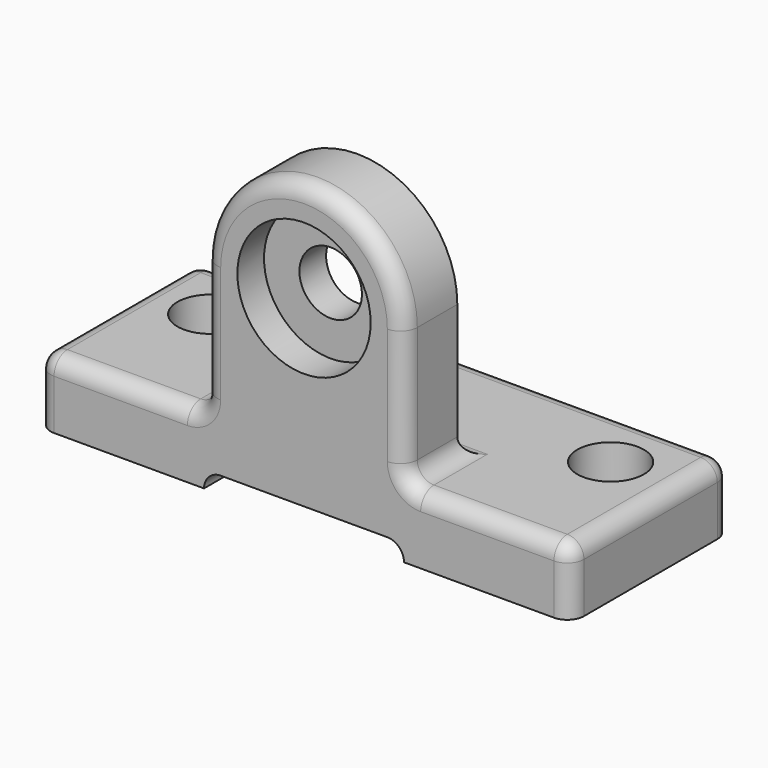
from build123d import *

# Parameters (mm, degrees)
F0_W           = 101.6
F0_H           = 38.1
F0_R           = 6.35
F1_DEPTH       = 12.7
F3_DEPTH       = 12.7
F4_D           = 11.90625
F4_CBORE_D     = 25.4
F4_CBORE_DEPTH = 6.35
F5_W           = 38.1
F5_H           = 3.175
F6_DEPTH       = 38.101
F9_R           = 3.175
F9_R_2         = 3.17499


# Not quite as in the source:
# - a fillet or chamfer is up to 0.001 mm smaller than in the source, because OpenCascade refuses the exact size
# - a feature of the source that left no trace in its solid (it failed there, or was rolled back) is left out
# - a length typed as a fraction of an inch, garbled in the dataset ("3 / 203.2 mm" for 3/8 in), is restored


with BuildPart() as f1:
    # F0 (on Top) → F1 (new body)
    with BuildSketch(Plane.XY):
        with Locations((12.3613710271, 3.3725141548)):
            Rectangle(F0_W, F0_H)
        with Locations((-25.7386289729, 9.7225141548)):
            Circle(F0_R, mode=Mode.SUBTRACT)
        with Locations((50.4613710271, 9.7225141548)):
            Circle(F0_R, mode=Mode.SUBTRACT)
    extrude(amount=F1_DEPTH)

    # F2 (on face) → F3 (join)
    with BuildSketch(Plane.XZ.offset(15.6774858452)):
        with BuildLine():
            Line((-6.6886289729, 38.1), (-6.6886289729, 12.7))
            Line((-6.6886289729, 12.7), (31.4113710271, 12.7))
            Line((31.4113710271, 12.7), (31.4113710271, 38.1))
            ThreePointArc((31.4113710271, 38.1), (12.3613710271, 57.15), (-6.6886289729, 38.1))
        make_face()
    extrude(amount=-F3_DEPTH)

    # F4 (through all)
    with Locations(Plane.XZ.offset(15.6774858452)):
        with Locations((12.3613710271, 38.1)):
            CounterBoreHole(F4_D / 2, F4_CBORE_D / 2, F4_CBORE_DEPTH)

    # F5 (on face) → F6 (cut, through all)
    with BuildSketch(Plane(origin=(0, 22.4225141548, 0), x_dir=(-1, 0, 0), z_dir=(0, 1, 0))):
        with Locations((-12.3613710271, 1.5875)):
            Rectangle(F5_W, F5_H)
    extrude(amount=-F6_DEPTH, mode=Mode.SUBTRACT)

    # F8: union 

    # F9 (call 1 of 3: OpenCascade refuses the feature's edges together)
    f9_edges = [f1.edges().sort_by_distance(p)[0] for p in [
        (63.161371, -15.677486, 6.35),
        (63.161371, 22.422514, 6.35),
        (-38.438629, -15.677486, 6.35),
        (-38.438629, 22.422514, 6.35),
        (12.361371, 22.422514, 12.7),
        (63.161371, 3.372514, 12.7),
        (-38.438629, 3.372514, 12.7),
        (47.286371, -15.677486, 12.7),
        (-22.563629, -15.677486, 12.7),
        (12.361371, -2.977486, 12.7),
        (31.411371, -9.327486, 12.7),
        (-6.688629, -9.327486, 12.7),
        (31.411371, -15.677486, 25.4),
        (12.361371, -15.677486, 57.15),
        (-6.688629, -15.677486, 25.4),
    ]]
    fillet(f9_edges, radius=F9_R)

    # F9#2 (call 2 of 3) (radius 3.175 in the source; OpenCascade refuses exactly that, so slightly less here)
    f9_2_edges = [f1.edges().sort_by_distance(p)[0] for p in [
        (-6.688629, 3.372514, 3.175),
    ]]
    fillet(f9_2_edges, radius=F9_R_2)

    # F9#3 (call 3 of 3) (radius 3.175 in the source; OpenCascade refuses exactly that, so slightly less here)
    f9_3_edges = [f1.edges().sort_by_distance(p)[0] for p in [
        (31.411371, 3.372514, 3.175),
    ]]
    fillet(f9_3_edges, radius=F9_R_2)


solid = f1.part
